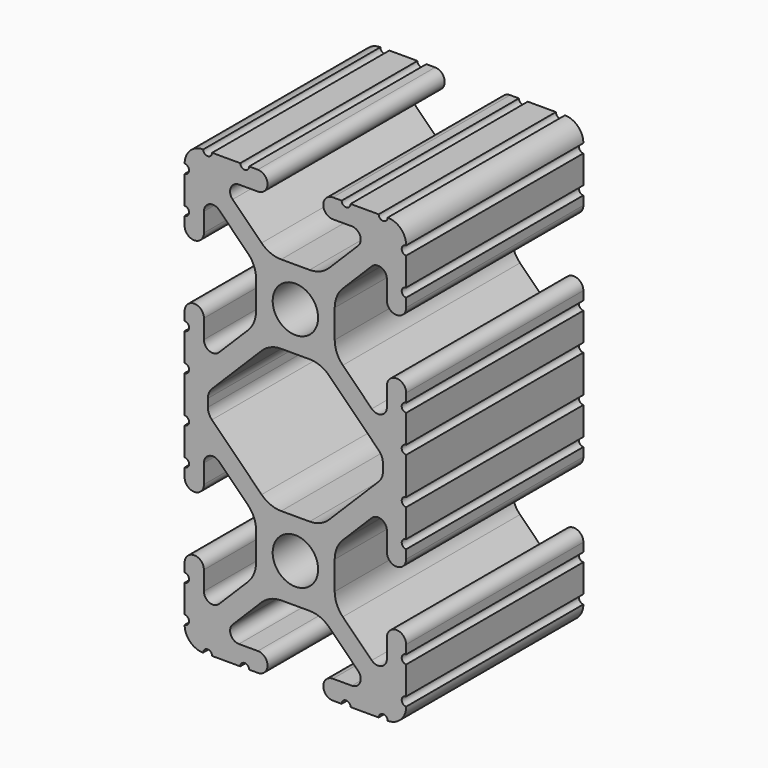
from build123d import *

# Parameters (mm, degrees)
F1_DEPTH = 25.4


# Not quite as in the source:
# - ends of sketch curves that miss each other by under 0.0002 mm in the source are joined


with BuildPart() as f1:
    # F0 (on Front) → F1 (new body)
    with BuildSketch(Plane.XZ):
        with BuildLine():
            ThreePointArc((-12.6999998568, 23.2791116031), (-12.1919492, 22.76475), (-12.6999998568, 22.2503883969))
            Line((-12.6999998568, 22.2503883969), (-12.7, 19.0246))
            ThreePointArc((-12.7, 19.0246), (-12.192, 18.5166), (-12.7, 18.0086))
            Line((-12.7, 18.0086), (-12.7, 17.0023028))
            ThreePointArc((-12.7, 17.0023028), (-11.5951, 15.8974028), (-10.4902, 17.0023028))
            Line((-10.4902, 17.0023028), (-10.4902, 19.1747902))
            ThreePointArc((-10.4902, 19.1747902), (-9.8630063673, 20.113451805), (-8.7557795103, 19.8932106897))
            Line((-8.7557795103, 19.8932106897), (-5.4384448, 16.5758622))
            ThreePointArc((-5.4384448, 16.5758622), (-4.7501824843, 15.5458268978), (-4.5085, 14.330807))
            Line((-4.5085, 14.330807), (-4.5085, 11.069193))
            ThreePointArc((-4.5085, 11.069193), (-4.7501824843, 9.8541731022), (-5.4384359697, 8.8241289697))
            Line((-5.4384359697, 8.8241289697), (-8.7557864, 5.5067962))
            ThreePointArc((-8.7557864, 5.5067962), (-9.8630063673, 5.286548195), (-10.4902, 6.2252098))
            Line((-10.4902, 6.2252098), (-10.4902, 8.3976972))
            ThreePointArc((-10.4902, 8.3976972), (-11.5951, 9.5025972), (-12.7, 8.3976972))
            Line((-12.7, 8.3976972), (-12.7, 7.3914))
            ThreePointArc((-12.7, 7.3914), (-12.192, 6.8834), (-12.7, 6.3754))
            Line((-12.7, 6.3754), (-12.7, 3.1496))
            ThreePointArc((-12.7, 3.1496), (-12.192, 2.6416), (-12.7, 2.1336))
            Line((-12.7, 2.1336), (-12.7, -2.1336))
            ThreePointArc((-12.7, -2.1336), (-12.192, -2.6416), (-12.7, -3.1496))
            Line((-12.7, -3.1496), (-12.7, -6.3754))
            ThreePointArc((-12.7, -6.3754), (-12.192, -6.8834), (-12.7, -7.3914))
            Line((-12.7, -7.3914), (-12.7, -8.3976972))
            ThreePointArc((-12.7, -8.3976972), (-11.5951, -9.5025972), (-10.4902, -8.3976972))
            Line((-10.4902, -8.3976972), (-10.4902, -6.2252098))
            ThreePointArc((-10.4902, -6.2252098), (-9.8630063673, -5.286548195), (-8.7557795103, -5.5067893103))
            Line((-8.7557795103, -5.5067893103), (-5.4384448, -8.8241378))
            ThreePointArc((-5.4384448, -8.8241378), (-4.7501824843, -9.8541731022), (-4.5085, -11.069193))
            Line((-4.5085, -11.069193), (-4.5085, -14.330807))
            ThreePointArc((-4.5085, -14.330807), (-4.7501824843, -15.5458268978), (-5.4384359697, -16.5758710303))
            Line((-5.4384359697, -16.5758710303), (-8.7557864, -19.8932038))
            ThreePointArc((-8.7557864, -19.8932038), (-9.8630063673, -20.113451805), (-10.4902, -19.1747902))
            Line((-10.4902, -19.1747902), (-10.4902, -17.0023028))
            ThreePointArc((-10.4902, -17.0023028), (-11.5951, -15.8974028), (-12.7, -17.0023028))
            Line((-12.7, -17.0023028), (-12.7, -18.0086))
            ThreePointArc((-12.7, -18.0086), (-12.192, -18.5166), (-12.7, -19.0246))
            Line((-12.7, -19.0246), (-12.7, -22.2504))
            ThreePointArc((-12.7, -22.2504), (-12.1919492, -22.76475), (-12.6999998568, -23.2791116031))
            ThreePointArc((-12.6999998568, -23.2791116031), (-12.0825733161, -24.7825733161), (-10.579099926, -25.4000122396))
            ThreePointArc((-10.579099926, -25.4000122396), (-10.06475, -24.8919492), (-9.5503883969, -25.3999998568))
            Line((-9.5503883969, -25.3999998568), (-6.3246, -25.4))
            ThreePointArc((-6.3246, -25.4), (-5.8166, -24.892), (-5.3086, -25.4))
            Line((-5.3086, -25.4), (-4.3023028, -25.4))
            ThreePointArc((-4.3023028, -25.4), (-3.1974028, -24.2951), (-4.3023028, -23.1902))
            Line((-4.3023028, -23.1902), (-6.4747902, -23.1902))
            ThreePointArc((-6.4747902, -23.1902), (-7.413451805, -22.5630063673), (-7.1932106897, -21.4557795103))
            Line((-7.1932106897, -21.4557795103), (-3.8758622, -18.1384448))
            ThreePointArc((-3.8758622, -18.1384448), (-2.8458268978, -17.4501824843), (-1.630807, -17.2085))
            Line((-1.630807, -17.2085), (1.630807, -17.2085))
            ThreePointArc((1.630807, -17.2085), (2.8458268978, -17.4501824843), (3.8758710303, -18.1384359697))
            Line((3.8758710303, -18.1384359697), (7.1932038, -21.4557864))
            ThreePointArc((7.1932038, -21.4557864), (7.413451805, -22.5630063673), (6.4747902, -23.1902))
            Line((6.4747902, -23.1902), (4.3023028, -23.1902))
            ThreePointArc((4.3023028, -23.1902), (3.1974028, -24.2951), (4.3023028, -25.4))
            Line((4.3023028, -25.4), (5.3086, -25.4))
            ThreePointArc((5.3086, -25.4), (5.8166, -24.892), (6.3246, -25.4))
            Line((6.3246, -25.4), (9.5504, -25.4))
            ThreePointArc((9.5504, -25.4), (10.06475, -24.8919492), (10.5791116031, -25.3999998568))
            ThreePointArc((10.5791116031, -25.3999998568), (12.0825733161, -24.7825733161), (12.7000122396, -23.279099926))
            ThreePointArc((12.7000122396, -23.279099926), (12.1919492, -22.76475), (12.6999998568, -22.2503883969))
            Line((12.6999998568, -22.2503883969), (12.7, -19.0246))
            ThreePointArc((12.7, -19.0246), (12.192, -18.5166), (12.7, -18.0086))
            Line((12.7, -18.0086), (12.7, -17.0023028))
            ThreePointArc((12.7, -17.0023028), (11.5951, -15.8974028), (10.4902, -17.0023028))
            Line((10.4902, -17.0023028), (10.4902, -19.1747902))
            ThreePointArc((10.4902, -19.1747902), (9.8630063673, -20.113451805), (8.7557795103, -19.8932106897))
            Line((8.7557795103, -19.8932106897), (5.4384448, -16.5758622))
            ThreePointArc((5.4384448, -16.5758622), (4.7501824843, -15.5458268978), (4.5085, -14.330807))
            Line((4.5085, -14.330807), (4.5085, -11.069193))
            ThreePointArc((4.5085, -11.069193), (4.7501824843, -9.8541731022), (5.4384359697, -8.8241289697))
            Line((5.4384359697, -8.8241289697), (8.7557864, -5.5067962))
            ThreePointArc((8.7557864, -5.5067962), (9.8630063673, -5.286548195), (10.4902, -6.2252098))
            Line((10.4902, -6.2252098), (10.4902, -8.3976972))
            ThreePointArc((10.4902, -8.3976972), (11.5951, -9.5025972), (12.7, -8.3976972))
            Line((12.7, -8.3976972), (12.7, -7.3914))
            ThreePointArc((12.7, -7.3914), (12.192, -6.8834), (12.7, -6.3754))
            Line((12.7, -6.3754), (12.7, -3.1496))
            ThreePointArc((12.7, -3.1496), (12.192, -2.6416), (12.7, -2.1336))
            Line((12.7, -2.1336), (12.7, 2.1336))
            ThreePointArc((12.7, 2.1336), (12.192, 2.6416), (12.7, 3.1496))
            Line((12.7, 3.1496), (12.7, 6.3754))
            ThreePointArc((12.7, 6.3754), (12.192, 6.8834), (12.7, 7.3914))
            Line((12.7, 7.3914), (12.7, 8.3976972))
            ThreePointArc((12.7, 8.3976972), (11.5951, 9.5025972), (10.4902, 8.3976972))
            Line((10.4902, 8.3976972), (10.4902, 6.2252098))
            ThreePointArc((10.4902, 6.2252098), (9.8630063673, 5.286548195), (8.7557795103, 5.5067893103))
            Line((8.7557795103, 5.5067893103), (5.4384448, 8.8241378))
            ThreePointArc((5.4384448, 8.8241378), (4.7501824843, 9.8541731022), (4.5085, 11.069193))
            Line((4.5085, 11.069193), (4.5085, 14.330807))
            ThreePointArc((4.5085, 14.330807), (4.7501824843, 15.5458268978), (5.4384359697, 16.5758710303))
            Line((5.4384359697, 16.5758710303), (8.7557864, 19.8932038))
            ThreePointArc((8.7557864, 19.8932038), (9.8630063673, 20.113451805), (10.4902, 19.1747902))
            Line((10.4902, 19.1747902), (10.4902, 17.0023028))
            ThreePointArc((10.4902, 17.0023028), (11.5951, 15.8974028), (12.7, 17.0023028))
            Line((12.7, 17.0023028), (12.7, 18.0086))
            ThreePointArc((12.7, 18.0086), (12.192, 18.5166), (12.7, 19.0246))
            Line((12.7, 19.0246), (12.7, 22.2504))
            ThreePointArc((12.7, 22.2504), (12.1919492, 22.76475), (12.6999998568, 23.2791116031))
            ThreePointArc((12.6999998568, 23.2791116031), (12.0825733161, 24.7825733161), (10.579099926, 25.4000122396))
            ThreePointArc((10.579099926, 25.4000122396), (10.06475, 24.8919492), (9.5503883969, 25.3999998568))
            Line((9.5503883969, 25.3999998568), (6.3246, 25.4))
            ThreePointArc((6.3246, 25.4), (5.8166, 24.892), (5.3086, 25.4))
            Line((5.3086, 25.4), (4.3023028, 25.4))
            ThreePointArc((4.3023028, 25.4), (3.1974028, 24.2951), (4.3023028, 23.1902))
            Line((4.3023028, 23.1902), (6.4747902, 23.1902))
            ThreePointArc((6.4747902, 23.1902), (7.413451805, 22.5630063673), (7.1932106897, 21.4557795103))
            Line((7.1932106897, 21.4557795103), (3.8758622, 18.1384448))
            ThreePointArc((3.8758622, 18.1384448), (2.8458268978, 17.4501824843), (1.630807, 17.2085))
            Line((1.630807, 17.2085), (-1.630807, 17.2085))
            ThreePointArc((-1.630807, 17.2085), (-2.8458268978, 17.4501824843), (-3.8758710303, 18.1384359697))
            Line((-3.8758710303, 18.1384359697), (-7.1932038, 21.4557864))
            ThreePointArc((-7.1932038, 21.4557864), (-7.413451805, 22.5630063673), (-6.4747902, 23.1902))
            Line((-6.4747902, 23.1902), (-4.3023028, 23.1902))
            ThreePointArc((-4.3023028, 23.1902), (-3.1974028, 24.2951), (-4.3023028, 25.4))
            Line((-4.3023028, 25.4), (-5.3086, 25.4))
            ThreePointArc((-5.3086, 25.4), (-5.8166, 24.892), (-6.3246, 25.4))
            Line((-6.3246, 25.4), (-9.5504, 25.4))
            ThreePointArc((-9.5504, 25.4), (-10.06475, 24.8919492), (-10.5791116031, 25.3999998568))
            ThreePointArc((-10.5791116031, 25.3999998568), (-12.0825733161, 24.7825733161), (-12.6999998568, 23.2791116031))
        make_face()
        with BuildLine():
            ThreePointArc((-2.6035, -12.7), (0, -10.0965), (2.6035, -12.7))
            ThreePointArc((2.6035, -12.7), (0, -15.3035), (-2.6035, -12.7))
        make_face(mode=Mode.SUBTRACT)
        with BuildLine():
            ThreePointArc((-10.033, 0.45212), (-9.9131254878, 1.0547698693), (-9.571751759, 1.565671759))
            Line((-9.571751759, 1.565671759), (-3.8758622, 7.2615552))
            ThreePointArc((-3.8758622, 7.2615552), (-2.8458268978, 7.9498175157), (-1.630807, 8.1915))
            Line((-1.630807, 8.1915), (1.630807, 8.1915))
            ThreePointArc((1.630807, 8.1915), (2.8458268978, 7.9498175157), (3.8758710303, 7.2615640303))
            Line((3.8758710303, 7.2615640303), (9.5717614, 1.5656814))
            ThreePointArc((9.5717614, 1.5656814), (9.9131254878, 1.0547698693), (10.033, 0.45212))
            Line((10.033, 0.45212), (10.033, -0.45212))
            ThreePointArc((10.033, -0.45212), (9.9131254878, -1.0547698693), (9.571751759, -1.565671759))
            Line((9.571751759, -1.565671759), (3.8758622, -7.2615552))
            ThreePointArc((3.8758622, -7.2615552), (2.8458268978, -7.9498175157), (1.630807, -8.1915))
            Line((1.630807, -8.1915), (-1.630807, -8.1915))
            ThreePointArc((-1.630807, -8.1915), (-2.8458268978, -7.9498175157), (-3.8758710303, -7.2615640303))
            Line((-3.8758710303, -7.2615640303), (-9.5717614, -1.5656814))
            ThreePointArc((-9.5717614, -1.5656814), (-9.9131254878, -1.0547698693), (-10.033, -0.45212))
            Line((-10.033, -0.45212), (-10.033, 0.45212))
        make_face(mode=Mode.SUBTRACT)
        with BuildLine():
            ThreePointArc((-2.6035, 12.7), (0, 15.3035), (2.6035, 12.7))
            ThreePointArc((2.6035, 12.7), (0, 10.0965), (-2.6035, 12.7))
        make_face(mode=Mode.SUBTRACT)
    extrude(amount=F1_DEPTH)


solid = f1.part
